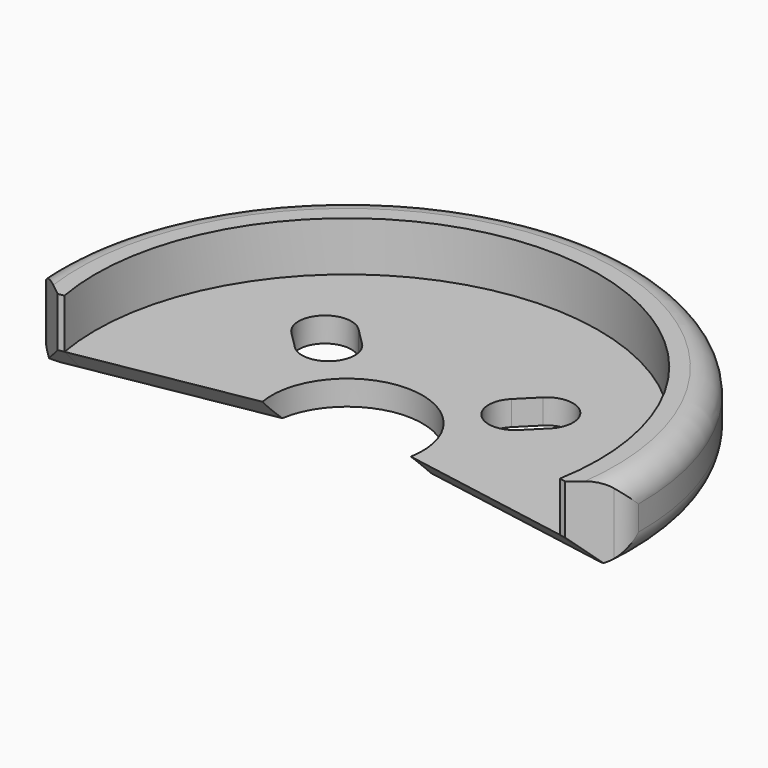
from build123d import *

# Parameters (mm, degrees)
F1_DEPTH    = 3
F2_DEPTH    = 1.5
F3_T1_DEPTH = 16.0790165437
F4_SIZE     = 1.49999
F5_T1_DEPTH = 8.1382032795
F5_T4_ANGLE = 209.6600935854
F5_T6_ANGLE = 209.6600935854


# Not quite as in the source:
# - a fillet or chamfer that OpenCascade refuses, or shapes differently, is made with other operations: its cross-section is extruded or revolved along the edge and cut away or added
# - a fillet or chamfer is up to 0.001 mm smaller than in the source, because OpenCascade refuses the exact size


with BuildPart() as f1:
    # F0 (on Top) → F1 (new body)
    with BuildSketch(Plane.XY):
        with BuildLine():
            Line((-17.480337616, -3.0822551536), (-15.0183182334, -2.6481347094))
            ThreePointArc((-15.0183182334, -2.6481347094), (0, 15.25), (15.0183182334, -2.6481347094))
            Line((15.0183182334, -2.6481347094), (17.480337616, -3.0822551536))
            ThreePointArc((17.480337616, -3.0822551536), (0, 17.75), (-17.480337616, -3.0822551536))
        make_face()
    extrude(amount=F1_DEPTH)

    # F0 (on Top) → F2 (join)
    with BuildSketch(Plane.XY):
        with BuildLine():
            Line((-17.480337616, -3.0822551536), (-15.0183182334, -2.6481347094))
            ThreePointArc((-15.0183182334, -2.6481347094), (0, 15.25), (15.0183182334, -2.6481347094))
            Line((15.0183182334, -2.6481347094), (17.480337616, -3.0822551536))
            ThreePointArc((17.480337616, -3.0822551536), (0, 17.75), (-17.480337616, -3.0822551536))
        make_face()
        with BuildLine():
            Line((-15.0183182334, -2.6481347094), (-4.5, -0.7934714132))
            ThreePointArc((-4.5, -0.7934714132), (0, 4.5694197535), (4.5, -0.7934714132))
            Line((4.5, -0.7934714132), (15.0183182334, -2.6481347094))
            ThreePointArc((15.0183182334, -2.6481347094), (0, 15.25), (-15.0183182334, -2.6481347094))
        make_face()
        with BuildLine():
            Line((-5.5861435714, 7.8488852712), (-4.5254833996, 6.7882250994))
            ThreePointArc((-4.5254833996, 6.7882250994), (-4.5254833996, 4.5254833996), (-6.7882250994, 4.5254833996))
            Line((-6.7882250994, 4.5254833996), (-7.8488852712, 5.5861435714))
            ThreePointArc((-7.8488852712, 5.5861435714), (-7.8488852712, 7.8488852712), (-5.5861435714, 7.8488852712))
        make_face(mode=Mode.SUBTRACT)
        with BuildLine():
            ThreePointArc((6.7882250994, 4.5254833996), (4.5254833996, 4.5254833996), (4.5254833996, 6.7882250994))
            Line((4.5254833996, 6.7882250994), (5.5861435714, 7.8488852712))
            ThreePointArc((5.5861435714, 7.8488852712), (7.8488852712, 7.8488852712), (7.8488852712, 5.5861435714))
            Line((7.8488852712, 5.5861435714), (6.7882250994, 4.5254833996))
        make_face(mode=Mode.SUBTRACT)
    extrude(amount=-F2_DEPTH)

    # F3: chamfer of 2 on 2 edges, made by hand

    # F3_s2 → F3_t1 (cut)
    with BuildSketch(Plane.XY.offset(-7.2895082718)):
        with BuildLine():
            Line((-15.3851589244, -2.7128186209), (-17.7302273788, -0.8375781136))
            ThreePointArc((-17.7302273788, -0.8375781136), (-17.6441291813, -1.935769985), (-17.480337616, -3.0822551536))
            Line((-17.480337616, -3.0822551536), (-15.3851589244, -2.7128186209))
        make_face()
        with BuildLine():
            Line((15.3851589244, -2.7128186209), (17.7302273788, -0.8375781136))
            ThreePointArc((17.7302273788, -0.8375781136), (17.6441291813, -1.935769985), (17.480337616, -3.0822551536))
            Line((17.480337616, -3.0822551536), (15.3851589244, -2.7128186209))
        make_face()
    extrude(amount=F3_T1_DEPTH, mode=Mode.SUBTRACT)

    # F4 (size 1.5 in the source; OpenCascade refuses exactly that, so slightly less here)
    f4_edges = [f1.edges().sort_by_distance(p)[0] for p in [
        (9.942579, -1.753145, -1.5),
        (-9.942579, -1.753145, -1.5),
    ]]
    chamfer(f4_edges, length=F4_SIZE)

    # F5: fillet of radius 1.5 on 4 edges, made by hand

    # F5_s2 → F5_t1 (cut)
    with BuildSketch(Plane.XY.offset(-3.3191016398)):
        with BuildLine():
            ThreePointArc((-17.7496579301, -0.1101969358), (-17.5995489023, -0.7550040841), (-17.1864813575, -1.2723861308))
            Line((-17.1864813575, -1.2723861308), (-17.7302273788, -0.8375781136))
            ThreePointArc((-17.7302273788, -0.8375781136), (-17.7436703144, -0.4739871018), (-17.7496579301, -0.1101969358))
        make_face()
        with BuildLine():
            ThreePointArc((17.1864813575, -1.2723861308), (17.5995489023, -0.7550040841), (17.7496579301, -0.1101969358))
            ThreePointArc((17.7496579301, -0.1101969358), (17.7436703144, -0.4739871018), (17.7302273788, -0.8375781136))
            Line((17.7302273788, -0.8375781136), (17.1864813575, -1.2723861308))
        make_face()
    extrude(amount=F5_T1_DEPTH, mode=Mode.SUBTRACT)

    # F5_s3 → F5_t4 (revolve, cut)
    with BuildSketch(Plane(origin=(0, 0, 0), x_dir=(0, 0, 1), z_dir=(-0.2559527399, -0.966689296, 0))):
        with BuildLine():
            ThreePointArc((3, -16.25), (2.5606601718, -17.3106601718), (1.5, -17.75))
            Line((1.5, -17.75), (3, -17.75))
            Line((3, -17.75), (3, -16.25))
        make_face()
    revolve(axis=Axis((0, 0, 3), (0, 0, 1)), revolution_arc=F5_T4_ANGLE, mode=Mode.SUBTRACT)

    # F5_s5 → F5_t6 (revolve, cut)
    with BuildSketch(Plane(origin=(0, 0, 0), x_dir=(0, 0, 1), z_dir=(-0.2559527399, -0.966689296, 0))):
        with BuildLine():
            ThreePointArc((-1.5, -16.25), (-1.0606601718, -17.3106601718), (0, -17.75))
            Line((0, -17.75), (-1.5, -17.75))
            Line((-1.5, -17.75), (-1.5, -16.25))
        make_face()
    revolve(axis=Axis((0, 0, -1.5), (0, 0, 1)), revolution_arc=F5_T6_ANGLE, mode=Mode.SUBTRACT)


solid = f1.part
